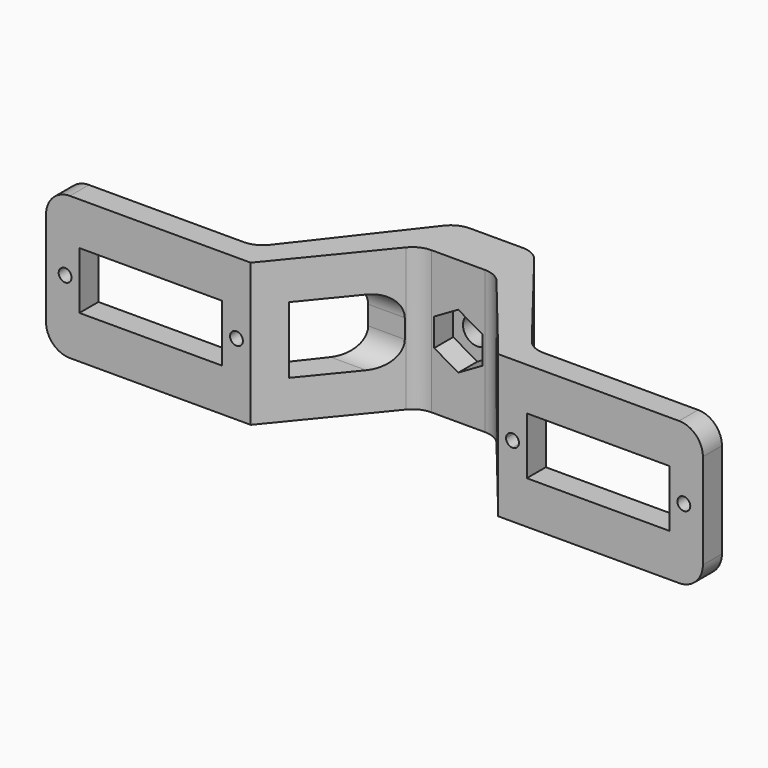
from build123d import *

# Parameters (mm, degrees)
F1_DEPTH = 30
F3_R     = 3
F4_DEPTH = 25
F5_DEPTH = 5
F6_W     = 15
F6_H     = 14
F7_DEPTH = 160
F8_R     = 5
F2_W     = 30
F2_H     = 12
F2_R     = 1.35
F9_DEPTH = 25


# Not quite as in the source:
# - a feature names something its author has since deleted; it is built from what else it names


with BuildPart() as f1:
    # F0 (on Top) → F1 (new body)
    with BuildSketch(Plane.XY):
        Polygon((29, 5), (8, 32), (-8, 32), (-29, 5), (-69, 5), (-69, 0), (-26, 0), (-8, 22), (8, 22), (26, 0), (69, 0), (69, 5), align=None)
    extrude(amount=F1_DEPTH)

    # F3 (on face) → F4 (cut)
    with BuildSketch(Plane.XZ.offset(-22)):
        with Locations((0, 15)):
            Circle(F3_R)
    extrude(amount=-F4_DEPTH, mode=Mode.SUBTRACT)

    # F3 (on face) → F5 (cut)
    with BuildSketch(Plane.XZ.offset(-22)):
        Polygon((0, 9.1687622812), (5.05, 12.0843811406), (5.05, 17.9156188594), (0, 20.8312377188), (-5.05, 17.9156188594), (-5.05, 12.0843811406), align=None)
        with Locations((0, 15)):
            Circle(F3_R, mode=Mode.SUBTRACT)
    extrude(amount=-F5_DEPTH, mode=Mode.SUBTRACT)

    # F6 (on face) → F7 (cut)
    with BuildSketch(Plane.YZ.offset(69)):
        with Locations((12.5, 15)):
            Rectangle(F6_W, F6_H)
    extrude(amount=-F7_DEPTH, mode=Mode.SUBTRACT)

    # F8
    f8_edges = [f1.edges().sort_by_distance(p)[0] for p in [
        (-8, 32, 15),
        (8, 32, 15),
        (-8, 22, 15),
        (8, 22, 15),
        (29, 5, 26),
        (29, 5, 4),
        (13.484848, 20, 8),
        (13.484848, 20, 22),
        (-13.484848, 20, 8),
        (-13.484848, 20, 22),
        (-29, 5, 4),
        (-29, 5, 26),
        (-69, 2.5, 30),
        (-69, 2.5, 0),
        (69, 2.5, 30),
        (69, 2.5, 0),
    ]]
    fillet(f8_edges, radius=F8_R)

    # F2 (on face) → F9 (cut)
    with BuildSketch(Plane(origin=(0, 5, 0), x_dir=(-1, 0, 0), z_dir=(0, 1, 0))):
        with Locations((47, 15)):
            Rectangle(F2_W, F2_H)
        with Locations((-47, 15)):
            Rectangle(F2_W, F2_H)
        with BuildLine():
            Line((-29, 13.65), (-29, 16.35))
            ThreePointArc((-29, 16.35), (-30.35, 15), (-29, 13.65))
        make_face()
        with BuildLine():
            ThreePointArc((-29, 13.65), (-28.0454058454, 14.0454058454), (-27.65, 15))
            ThreePointArc((-27.65, 15), (-28.0454058454, 15.9545941546), (-29, 16.35))
            Line((-29, 16.35), (-29, 13.65))
        make_face()
        with Locations((-65, 15)):
            Circle(F2_R)
        with Locations((29, 15)):
            Circle(F2_R)
        with Locations((65, 15)):
            Circle(F2_R)
    extrude(amount=-F9_DEPTH, mode=Mode.SUBTRACT)


solid = f1.part
